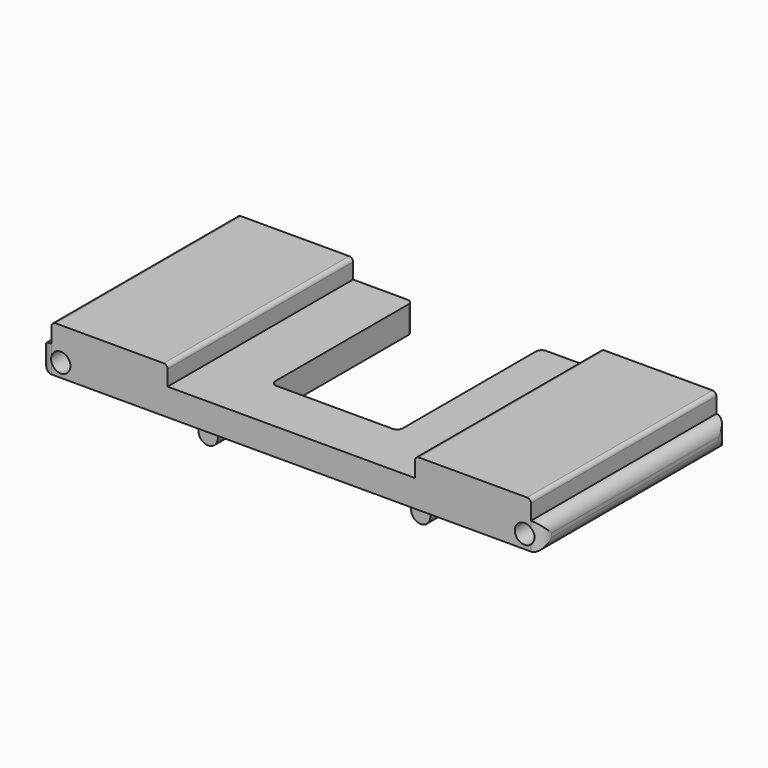
from build123d import *

# Parameters (mm, degrees)
F0_W        = 1300
F0_H        = 70
F1_DEPTH    = 600
F2_R        = 25
F3_DEPTH    = 800
F4_T1_DEPTH = 750
F4_T3_DEPTH = 220
F5_W        = 330
F5_H        = 460
F6_DEPTH    = 100
F7_R        = 15
F8_W        = 50
F8_H        = 50
F9_DEPTH    = 80
F10_R       = 24.99999
F11_R       = 20
F12_DEPTH   = 60
F13_R       = 20
F14_DEPTH   = 60
F15_R       = 20
F16_DEPTH   = 60
F17_R       = 20
F18_DEPTH   = 60
F19_W       = 300
F19_H       = 600
F20_DEPTH   = 50
F21_R       = 10
F23_DEPTH   = 10
F25_DEPTH   = 15
F26_R       = 10
F28_DEPTH   = 15
F30_DEPTH   = 15
F31_R       = 10
F31_2_R     = 10
F31_3_R     = 10


# Not quite as in the source:
# - a fillet or chamfer that OpenCascade refuses, or shapes differently, is made with other operations: its cross-section is extruded or revolved along the edge and cut away or added
# - a fillet or chamfer is up to 0.001 mm smaller than in the source, because OpenCascade refuses the exact size


with BuildPart() as f1:
    # F0 (on Front) → F1 (new body)
    with BuildSketch(Plane.XZ):
        with Locations((650, 35)):
            Rectangle(F0_W, F0_H)
    extrude(amount=F1_DEPTH)

    # F2 (on face) → F3 (cut)
    with BuildSketch(Plane.XZ.offset(600)):
        with Locations((53.6256714825, 34.9870798825)):
            Circle(F2_R)
        with Locations((1253.6256714825, 34.9870798825)):
            Circle(F2_R)
    extrude(amount=-F3_DEPTH, mode=Mode.SUBTRACT)

    # F4: fillet of radius 30 on 8 edges, made by hand

    # F4_s2 → F4_t1 (cut)
    with BuildSketch(Plane.XZ.offset(-75)):
        with BuildLine():
            ThreePointArc((0, 40), (8.7867965644, 61.2132034356), (30, 70))
            Line((30, 70), (0, 70))
            Line((0, 70), (0, 40))
        make_face()
        with BuildLine():
            ThreePointArc((0, 30), (8.7867965644, 8.7867965644), (30, 0))
            Line((30, 0), (0, 0))
            Line((0, 0), (0, 30))
        make_face()
        with BuildLine():
            ThreePointArc((1270, 0), (1291.2132034356, 8.7867965644), (1300, 30))
            Line((1300, 30), (1300, 0))
            Line((1300, 0), (1270, 0))
        make_face()
        with BuildLine():
            ThreePointArc((1270, 70), (1291.2132034356, 61.2132034356), (1300, 40))
            Line((1300, 40), (1300, 70))
            Line((1300, 70), (1270, 70))
        make_face()
    extrude(amount=F4_T1_DEPTH, mode=Mode.SUBTRACT)

    # F4_s4 → F4_t3 (cut)
    with BuildSketch(Plane.XY.offset(-75)):
        with BuildLine():
            ThreePointArc((0, -30), (8.7867965644, -8.7867965644), (30, 0))
            Line((30, 0), (0, 0))
            Line((0, 0), (0, -30))
        make_face()
        with BuildLine():
            ThreePointArc((0, -570), (8.7867965644, -591.2132034356), (30, -600))
            Line((30, -600), (0, -600))
            Line((0, -600), (0, -570))
        make_face()
        with BuildLine():
            ThreePointArc((1270, 0), (1291.2132034356, -8.7867965644), (1300, -30))
            Line((1300, -30), (1300, 0))
            Line((1300, 0), (1270, 0))
        make_face()
        with BuildLine():
            ThreePointArc((1270, -600), (1291.2132034356, -591.2132034356), (1300, -570))
            Line((1300, -570), (1300, -600))
            Line((1300, -600), (1270, -600))
        make_face()
    extrude(amount=F4_T3_DEPTH, mode=Mode.SUBTRACT)

    # F5 (on face) → F6 (cut)
    with BuildSketch(Plane.XY.offset(70)):
        with Locations((650, -230)):
            Rectangle(F5_W, F5_H)
    extrude(amount=-F6_DEPTH, mode=Mode.SUBTRACT)

    # F7
    f7_edges = [f1.edges().sort_by_distance(p)[0] for p in [
        (815, 0, 35),
        (485, 0, 35),
        (485, -460, 35),
        (815, -460, 35),
    ]]
    fillet(f7_edges, radius=F7_R)

    # F8 (on face) → F9 (join)
    with BuildSketch(Plane(origin=(0, 0, 0), x_dir=(1, 0, 0), z_dir=(0, 0, -1))):
        with Locations((375, 500)):
            Rectangle(F8_W, F8_H)
        with Locations((925, 500)):
            Rectangle(F8_W, F8_H)
        with Locations((975, 135)):
            Rectangle(F8_W, F8_H)
        with Locations((325, 135)):
            Rectangle(F8_W, F8_H)
    extrude(amount=F9_DEPTH)

    # F10 (radius 25 in the source; OpenCascade refuses exactly that, so slightly less here)
    f10_edges = [f1.edges().sort_by_distance(p)[0] for p in [
        (350, -500, -80),
        (400, -500, -80),
        (350, -135, -80),
        (300, -135, -80),
        (950, -500, -80),
        (900, -500, -80),
        (950, -135, -80),
        (1000, -135, -80),
    ]]
    fillet(f10_edges, radius=F10_R)

    # F11 (on face) → F12 (join)
    with BuildSketch(Plane(origin=(0, -110, 0), x_dir=(-1, 0, 0), z_dir=(0, 1, 0))):
        with Locations((-975, -55)):
            Circle(F11_R)
    extrude(amount=F12_DEPTH)

    # F13 (on face) → F14 (join)
    with BuildSketch(Plane(origin=(0, -110, 0), x_dir=(-1, 0, 0), z_dir=(0, 1, 0))):
        with Locations((-325, -55)):
            Circle(F13_R)
    extrude(amount=F14_DEPTH)

    # F15 (on face) → F16 (join)
    with BuildSketch(Plane(origin=(0, -475, 0), x_dir=(-1, 0, 0), z_dir=(0, 1, 0))):
        with Locations((-375, -55)):
            Circle(F15_R)
    extrude(amount=F16_DEPTH)

    # F17 (on face) → F18 (join)
    with BuildSketch(Plane(origin=(0, -475, 0), x_dir=(-1, 0, 0), z_dir=(0, 1, 0))):
        with Locations((-925, -55)):
            Circle(F17_R)
    extrude(amount=F18_DEPTH)

    # F19 (on face) → F20 (join)
    with BuildSketch(Plane.XY.offset(70)):
        with Locations((180, -300)):
            Rectangle(F19_W, F19_H)
        with Locations((1120, -300)):
            Rectangle(F19_W, F19_H)
    extrude(amount=F20_DEPTH)

    # F21
    f21_edges = [f1.edges().sort_by_distance(p)[0] for p in [
        (1270, -300, 120),
        (30, -300, 120),
        (330, -300, 120),
        (970, -300, 120),
    ]]
    fillet(f21_edges, radius=F21_R)


with BuildPart() as f23:
    # F22 (on face) → F23 (new body)
    with BuildSketch(Plane(origin=(0, -50, 0), x_dir=(-1, 0, 0), z_dir=(0, 1, 0))):
        with BuildLine():
            Line((-995, -25), (-995, -55))
            ThreePointArc((-995, -55), (-975, -35), (-955, -55))
            Line((-955, -55), (-955, -25))
            Line((-955, -25), (-995, -25))
        make_face()
    extrude(amount=-F23_DEPTH)

    # F26
    f26_edges = [f23.edges().sort_by_distance(p)[0] for p in [
        (995, -55, -25),
        (955, -55, -25),
    ]]
    fillet(f26_edges, radius=F26_R)


with BuildPart() as f25:
    # F24 (on face) → F25 (new body)
    with BuildSketch(Plane(origin=(0, -415, 0), x_dir=(-1, 0, 0), z_dir=(0, 1, 0))):
        with BuildLine():
            Line((-945, -25), (-945, -55))
            ThreePointArc((-945, -55), (-925, -35), (-905, -55))
            Line((-905, -55), (-905, -25))
            Line((-905, -25), (-945, -25))
        make_face()
    extrude(amount=-F25_DEPTH)

    # F31
    f31_edges = [f25.edges().sort_by_distance(p)[0] for p in [
        (905, -422.5, -25),
        (945, -422.5, -25),
    ]]
    fillet(f31_edges, radius=F31_R)


with BuildPart() as f28:
    # F27 (on face) → F28 (new body)
    with BuildSketch(Plane(origin=(0, -50, 0), x_dir=(-1, 0, 0), z_dir=(0, 1, 0))):
        with BuildLine():
            Line((-345, -25), (-345, -55))
            ThreePointArc((-345, -55), (-325, -35), (-305, -55))
            Line((-305, -55), (-305, -25))
            Line((-305, -25), (-345, -25))
        make_face()
    extrude(amount=-F28_DEPTH)

    # F31#2
    f31_2_edges = [f28.edges().sort_by_distance(p)[0] for p in [
        (345, -57.5, -25),
        (305, -57.5, -25),
    ]]
    fillet(f31_2_edges, radius=F31_2_R)


with BuildPart() as f30:
    # F29 (on face) → F30 (new body)
    with BuildSketch(Plane(origin=(0, -415, 0), x_dir=(-1, 0, 0), z_dir=(0, 1, 0))):
        with BuildLine():
            Line((-395, -25), (-395, -55))
            ThreePointArc((-395, -55), (-375, -35), (-355, -55))
            Line((-355, -55), (-355, -25))
            Line((-355, -25), (-395, -25))
        make_face()
    extrude(amount=-F30_DEPTH)

    # F31#3
    f31_3_edges = [f30.edges().sort_by_distance(p)[0] for p in [
        (395, -422.5, -25),
        (355, -422.5, -25),
    ]]
    fillet(f31_3_edges, radius=F31_3_R)


solid = Compound([f1.part, f23.part, f25.part, f28.part, f30.part])
